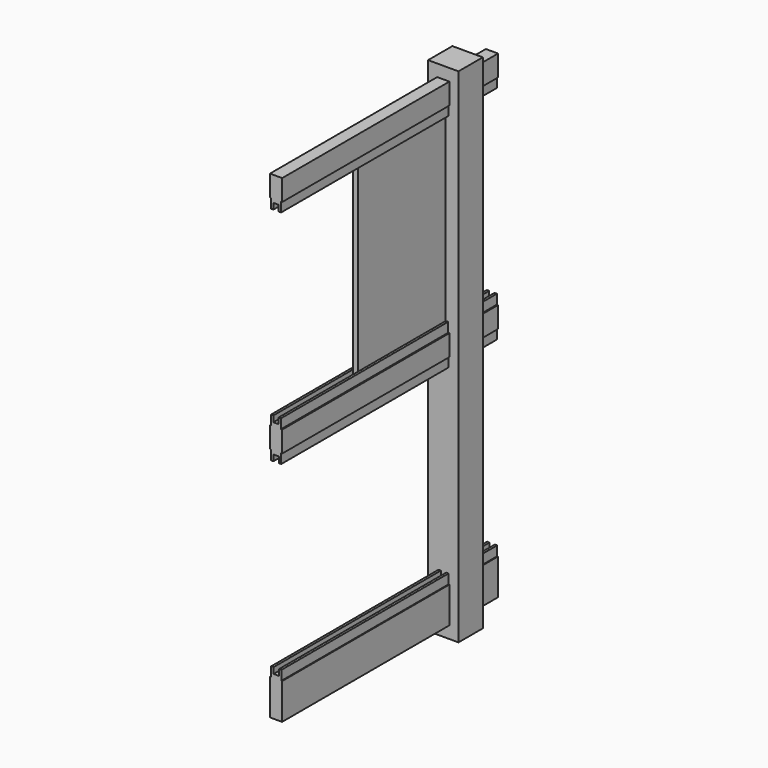
from build123d import *

# Parameters (mm, degrees)
F0_W          = 127
F0_H          = 2100
F1_DEPTH      = 127
F2_DEPTH      = 127
F2_DEPTH_BACK = 1000
F0_W_2        = 10.0161342862
F0_H_2        = 803.2517696619
F3_DEPTH      = 586


with BuildPart() as f1:
    # F0 (on Front) → F1 (new body)
    with BuildSketch(Plane.XZ):
        Rectangle(F0_W, F0_H)
        Polygon((-10.3423068728, -835), (0.7857291494, -835), (11.9137651715, -835), (11.9137651715, -810), (21.7857291494, -810), (21.7857291494, -850), (25, -850), (25, -1000), (-25, -1000), (-25, -850), (-20.2142708506, -850), (-20.2142708506, -810), (-10.3423068728, -810), align=None, mode=Mode.SUBTRACT)
        Polygon((-10.0161342919, 895.125884831), (-2.774e-07, 895.125884831), (10.0161340088, 895.125884831), (10.0161340088, 91.874115169), (-5.7e-09, 91.874115169), (-10.0161342919, 91.874115169), align=None, mode=Mode.SUBTRACT)
        Polygon((-11.5747122988, 90), (-5.1e-09, 90), (10.6813597456, 90), (10.6813597456, 115), (20.5533237234, 115), (20.5533237234, 75), (25.5, 75), (25.5, -13), (21.3999971747, -13), (21.3999971747, -53), (11.5280331969, -53), (11.5280331969, -28), (0.7857291494, -28), (-10.7280388474, -28), (-10.7280388474, -53), (-20.6000028253, -53), (-20.6000028253, -13), (-25.5, -13), (-25.5, 75), (-21.4466762766, 75), (-21.4466762766, 115), (-11.5747122988, 115), align=None, mode=Mode.SUBTRACT)
        Polygon((25.5, 1000), (25.5, 912), (20.9999997169, 912), (20.9999997169, 872), (11.1280357391, 872), (11.1280357391, 897), (-2.78e-07, 897), (-11.1280363053, 897), (-11.1280363053, 872), (-21.0000002831, 872), (-21.0000002831, 912), (-25.5, 912), (-25.5, 1000), align=None, mode=Mode.SUBTRACT)
        Polygon((20.9999997169, 872), (20.9999997169, 912), (-2.831e-07, 912), (-2.78e-07, 897), (11.1280357391, 897), (11.1280357391, 872), align=None)
        Polygon((-2.78e-07, 897), (-2.831e-07, 912), (-21.0000002831, 912), (-21.0000002831, 872), (-11.1280363053, 872), (-11.1280363053, 897), align=None)
        Polygon((21.3999971747, -53), (21.3999971747, -13), (0.7857291494, -13), (0.7857291494, -28), (11.5280331969, -28), (11.5280331969, -53), align=None)
        Polygon((0.7857291494, -13), (-20.6000028253, -13), (-20.6000028253, -53), (-10.7280388474, -53), (-10.7280388474, -28), (0.7857291494, -28), align=None)
    extrude(amount=F1_DEPTH)

    # F0 (on Front) → F2 (join, two sides)
    with BuildSketch(Plane.XZ) as f2_sk:
        Polygon((11.9137651715, -835), (0.7857291494, -835), (0.7857291494, -850), (21.7857291494, -850), (21.7857291494, -810), (11.9137651715, -810), align=None)
        Polygon((0.7857291494, -850), (0.7857291494, -835), (-10.3423068728, -835), (-10.3423068728, -810), (-20.2142708506, -810), (-20.2142708506, -850), align=None)
        Polygon((10.6813597456, 90), (-5.1e-09, 90), (0, 75), (20.5533237234, 75), (20.5533237234, 115), (10.6813597456, 115), align=None)
        Polygon((0, 75), (-5.1e-09, 90), (-11.5747122988, 90), (-11.5747122988, 115), (-21.4466762766, 115), (-21.4466762766, 75), align=None)
        Polygon((20.9999997169, 912), (25.5, 912), (25.5, 1000), (-25.5, 1000), (-25.5, 912), (-21.0000002831, 912), (-2.831e-07, 912), align=None)
        Polygon((20.9999997169, 872), (20.9999997169, 912), (-2.831e-07, 912), (-2.78e-07, 897), (11.1280357391, 897), (11.1280357391, 872), align=None)
        Polygon((-2.78e-07, 897), (-2.831e-07, 912), (-21.0000002831, 912), (-21.0000002831, 872), (-11.1280363053, 872), (-11.1280363053, 897), align=None)
        Polygon((20.5533237234, 75), (0, 75), (-21.4466762766, 75), (-25.5, 75), (-25.5, -13), (-20.6000028253, -13), (0.7857291494, -13), (21.3999971747, -13), (25.5, -13), (25.5, 75), align=None)
        Polygon((21.3999971747, -53), (21.3999971747, -13), (0.7857291494, -13), (0.7857291494, -28), (11.5280331969, -28), (11.5280331969, -53), align=None)
        Polygon((0.7857291494, -13), (-20.6000028253, -13), (-20.6000028253, -53), (-10.7280388474, -53), (-10.7280388474, -28), (0.7857291494, -28), align=None)
        Polygon((21.7857291494, -850), (0.7857291494, -850), (-20.2142708506, -850), (-25, -850), (-25, -1000), (25, -1000), (25, -850), align=None)
    extrude(amount=-F2_DEPTH)
    extrude(f2_sk.sketch, amount=F2_DEPTH_BACK)

    # F0 (on Front) → F3 (join)
    with BuildSketch(Plane.XZ):
        with Locations((5.0080668657, 493.5)):
            Rectangle(F0_W_2, F0_H_2)
        with Locations((-5.0080671488, 493.5)):
            Rectangle(F0_W_2, F0_H_2)
    extrude(amount=F3_DEPTH)


solid = f1.part
